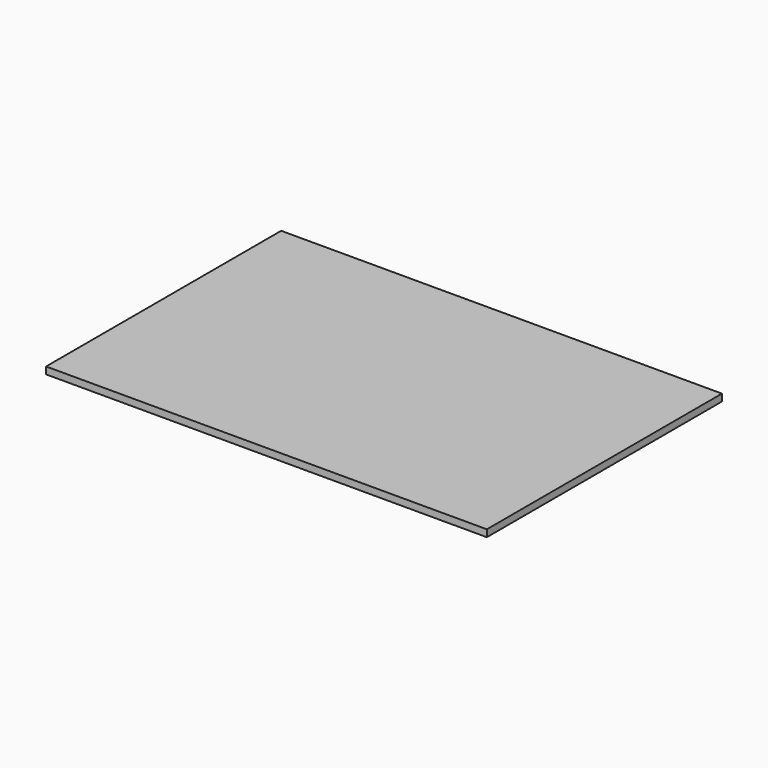
from build123d import *

# Parameters (mm, degrees)
F0_W     = 38.1
F0_H     = 2057.4
F0_H_2   = 114.3
F0_W_2   = 330.2
F0_W_3   = 552.45
F0_H_3   = 1752.6
F0_W_4   = 590.55
F1_DEPTH = 12.7
F2_DEPTH = 38.1


with BuildPart() as f1:
    # F0 (on Top) → F1 (new body)
    with BuildSketch(Plane.XY):
        Polygon((1600.2, 1028.7), (1600.2, 1066.8), (838.2, 1066.8), (838.2, 1028.7), (1193.8, 1028.7), (1231.9, 1028.7), (1562.1, 1028.7), align=None)
        Polygon((838.2, 1028.7), (838.2, 1066.8), (-381, 1066.8), (-1600.2, 1066.8), (-1600.2, 1028.7), (-1562.1, 1028.7), (-971.55, 1028.7), (-933.45, 1028.7), (-381, 1028.7), (-342.9, 1028.7), (209.55, 1028.7), (247.65, 1028.7), (800.1, 1028.7), align=None)
        with Locations((1581.15, 0)):
            Rectangle(F0_W, F0_H)
        Polygon((1193.8, 1028.7), (838.2, 1028.7), (838.2, 914.4), (838.2, 876.3), (838.2, -876.3), (838.2, -914.4), (838.2, -1028.7), (1193.8, -1028.7), align=None)
        with Locations((819.15, 971.55)):
            Rectangle(F0_W, F0_H_2)
        Polygon((1600.2, -1066.8), (1600.2, -1028.7), (1562.1, -1028.7), (1231.9, -1028.7), (1193.8, -1028.7), (838.2, -1028.7), (800.1, -1028.7), (247.65, -1028.7), (209.55, -1028.7), (-342.9, -1028.7), (-381, -1028.7), (-381, -1066.8), align=None)
        with Locations((1397, 0)):
            Rectangle(F0_W_2, F0_H)
        Polygon((838.2, 876.3), (838.2, 914.4), (800.1, 914.4), (247.65, 914.4), (209.55, 914.4), (-342.9, 914.4), (-381, 914.4), (-933.45, 914.4), (-971.55, 914.4), (-1562.1, 914.4), (-1600.2, 914.4), (-1600.2, 876.3), (-1562.1, 876.3), (-971.55, 876.3), (-933.45, 876.3), (-381, 876.3), (-342.9, 876.3), (209.55, 876.3), (247.65, 876.3), (800.1, 876.3), align=None)
        with Locations((523.875, 971.55)):
            Rectangle(F0_W_3, F0_H_2)
        with Locations((1212.85, 0)):
            Rectangle(F0_W, F0_H)
        with Locations((-1581.15, 971.55)):
            Rectangle(F0_W, F0_H_2)
        with Locations((819.15, 0)):
            Rectangle(F0_W, F0_H_3)
        with Locations((228.6, 971.55)):
            Rectangle(F0_W, F0_H_2)
        Polygon((-1600.2, -1066.8), (-381, -1066.8), (-381, -1028.7), (-933.45, -1028.7), (-971.55, -1028.7), (-1562.1, -1028.7), (-1600.2, -1028.7), align=None)
        with Locations((-1266.825, 971.55)):
            Rectangle(F0_W_4, F0_H_2)
        Polygon((838.2, -914.4), (838.2, -876.3), (800.1, -876.3), (247.65, -876.3), (209.55, -876.3), (-342.9, -876.3), (-381, -876.3), (-933.45, -876.3), (-971.55, -876.3), (-1562.1, -876.3), (-1600.2, -876.3), (-1600.2, -914.4), (-1562.1, -914.4), (-971.55, -914.4), (-933.45, -914.4), (-381, -914.4), (-342.9, -914.4), (209.55, -914.4), (247.65, -914.4), (800.1, -914.4), align=None)
        with Locations((523.875, 0)):
            Rectangle(F0_W_3, F0_H_3)
        with Locations((-66.675, 971.55)):
            Rectangle(F0_W_3, F0_H_2)
        with Locations((819.15, -971.55)):
            Rectangle(F0_W, F0_H_2)
        with Locations((-361.95, -971.55)):
            Rectangle(F0_W, F0_H_2)
        with Locations((-657.225, -971.55)):
            Rectangle(F0_W_3, F0_H_2)
        with Locations((-1581.15, 0)):
            Rectangle(F0_W, F0_H_3)
        with Locations((-952.5, 971.55)):
            Rectangle(F0_W, F0_H_2)
        with Locations((228.6, 0)):
            Rectangle(F0_W, F0_H_3)
        with Locations((-361.95, 971.55)):
            Rectangle(F0_W, F0_H_2)
        with Locations((523.875, -971.55)):
            Rectangle(F0_W_3, F0_H_2)
        with Locations((-1581.15, -971.55)):
            Rectangle(F0_W, F0_H_2)
        with Locations((-952.5, -971.55)):
            Rectangle(F0_W, F0_H_2)
        with Locations((-66.675, -971.55)):
            Rectangle(F0_W_3, F0_H_2)
        with Locations((-1266.825, 0)):
            Rectangle(F0_W_4, F0_H_3)
        with Locations((-657.225, 971.55)):
            Rectangle(F0_W_3, F0_H_2)
        with Locations((-66.675, 0)):
            Rectangle(F0_W_3, F0_H_3)
        with Locations((228.6, -971.55)):
            Rectangle(F0_W, F0_H_2)
        with Locations((-1266.825, -971.55)):
            Rectangle(F0_W_4, F0_H_2)
        with Locations((-952.5, 0)):
            Rectangle(F0_W, F0_H_3)
        with Locations((-361.95, 0)):
            Rectangle(F0_W, F0_H_3)
        with Locations((-657.225, 0)):
            Rectangle(F0_W_3, F0_H_3)
    extrude(amount=F1_DEPTH)

    # F0 (on Top) → F2 (join)
    with BuildSketch(Plane.XY):
        Polygon((1600.2, 1028.7), (1600.2, 1066.8), (838.2, 1066.8), (838.2, 1028.7), (1193.8, 1028.7), (1231.9, 1028.7), (1562.1, 1028.7), align=None)
        Polygon((838.2, 1028.7), (838.2, 1066.8), (-381, 1066.8), (-1600.2, 1066.8), (-1600.2, 1028.7), (-1562.1, 1028.7), (-971.55, 1028.7), (-933.45, 1028.7), (-381, 1028.7), (-342.9, 1028.7), (209.55, 1028.7), (247.65, 1028.7), (800.1, 1028.7), align=None)
        with Locations((1581.15, 0)):
            Rectangle(F0_W, F0_H)
        with Locations((819.15, 971.55)):
            Rectangle(F0_W, F0_H_2)
        Polygon((1600.2, -1066.8), (1600.2, -1028.7), (1562.1, -1028.7), (1231.9, -1028.7), (1193.8, -1028.7), (838.2, -1028.7), (800.1, -1028.7), (247.65, -1028.7), (209.55, -1028.7), (-342.9, -1028.7), (-381, -1028.7), (-381, -1066.8), align=None)
        Polygon((838.2, 876.3), (838.2, 914.4), (800.1, 914.4), (247.65, 914.4), (209.55, 914.4), (-342.9, 914.4), (-381, 914.4), (-933.45, 914.4), (-971.55, 914.4), (-1562.1, 914.4), (-1600.2, 914.4), (-1600.2, 876.3), (-1562.1, 876.3), (-971.55, 876.3), (-933.45, 876.3), (-381, 876.3), (-342.9, 876.3), (209.55, 876.3), (247.65, 876.3), (800.1, 876.3), align=None)
        with Locations((1212.85, 0)):
            Rectangle(F0_W, F0_H)
        with Locations((-1581.15, 971.55)):
            Rectangle(F0_W, F0_H_2)
        with Locations((819.15, 0)):
            Rectangle(F0_W, F0_H_3)
        with Locations((228.6, 971.55)):
            Rectangle(F0_W, F0_H_2)
        Polygon((-1600.2, -1066.8), (-381, -1066.8), (-381, -1028.7), (-933.45, -1028.7), (-971.55, -1028.7), (-1562.1, -1028.7), (-1600.2, -1028.7), align=None)
        Polygon((838.2, -914.4), (838.2, -876.3), (800.1, -876.3), (247.65, -876.3), (209.55, -876.3), (-342.9, -876.3), (-381, -876.3), (-933.45, -876.3), (-971.55, -876.3), (-1562.1, -876.3), (-1600.2, -876.3), (-1600.2, -914.4), (-1562.1, -914.4), (-971.55, -914.4), (-933.45, -914.4), (-381, -914.4), (-342.9, -914.4), (209.55, -914.4), (247.65, -914.4), (800.1, -914.4), align=None)
        with Locations((819.15, -971.55)):
            Rectangle(F0_W, F0_H_2)
        with Locations((-361.95, -971.55)):
            Rectangle(F0_W, F0_H_2)
        with Locations((-1581.15, 0)):
            Rectangle(F0_W, F0_H_3)
        with Locations((-952.5, 971.55)):
            Rectangle(F0_W, F0_H_2)
        with Locations((228.6, 0)):
            Rectangle(F0_W, F0_H_3)
        with Locations((-361.95, 971.55)):
            Rectangle(F0_W, F0_H_2)
        with Locations((-1581.15, -971.55)):
            Rectangle(F0_W, F0_H_2)
        with Locations((-952.5, -971.55)):
            Rectangle(F0_W, F0_H_2)
        with Locations((228.6, -971.55)):
            Rectangle(F0_W, F0_H_2)
        with Locations((-952.5, 0)):
            Rectangle(F0_W, F0_H_3)
        with Locations((-361.95, 0)):
            Rectangle(F0_W, F0_H_3)
    extrude(amount=-F2_DEPTH)


solid = f1.part
